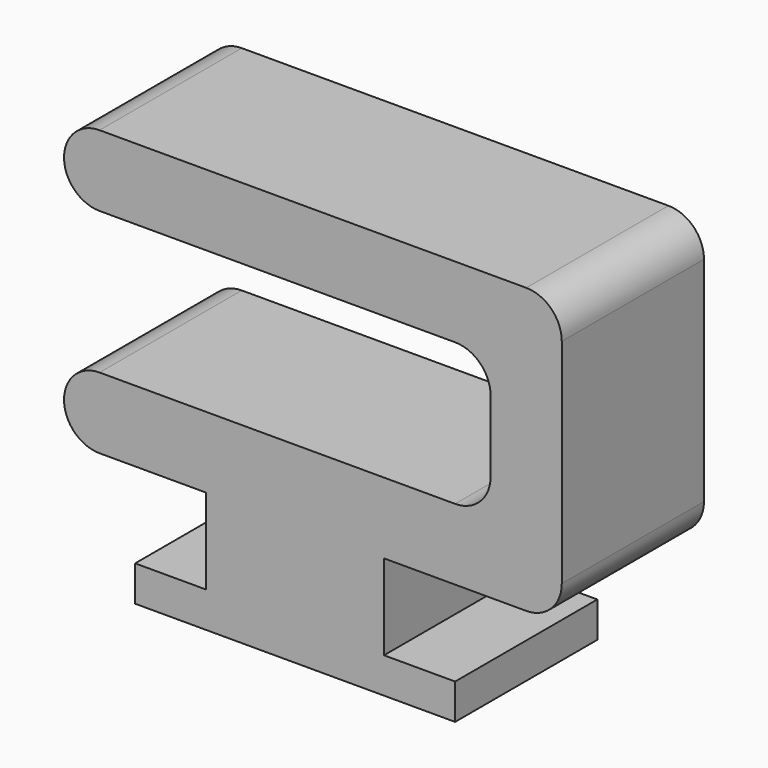
from build123d import *

# Parameters (mm, degrees)
F1_DEPTH = 5
F2_R     = 0.99999


# Not quite as in the source:
# - a fillet or chamfer is up to 0.001 mm smaller than in the source, because OpenCascade refuses the exact size
# - a feature names something its author has since deleted; it is built from what else it names


with BuildPart() as f1:
    # F0 (on Front) → F1 (new body)
    with BuildSketch(Plane.XZ):
        Polygon((-4, 0), (0, 0), (0, -2.4), (-2, -2.4), (-2, -3.4), (7, -3.4), (7, -2.4), (5, -2.4), (5, 0), (10, 0), (10, 8), (-4, 8), (-4, 6), (8, 6), (8, 2), (-4, 2), align=None)
    extrude(amount=F1_DEPTH)

    # F2 (radius 1 in the source; OpenCascade refuses exactly that, so slightly less here)
    f2_edges = [f1.edges().sort_by_distance(p)[0] for p in [
        (8, -2.5, 6),
        (8, -2.5, 2),
        (10, -2.5, 0),
        (10, -2.5, 8),
        (-4, -2.5, 8),
        (-4, -2.5, 6),
        (-4, -2.5, 0),
        (-4, -2.5, 2),
    ]]
    fillet(f2_edges, radius=F2_R)


solid = f1.part
